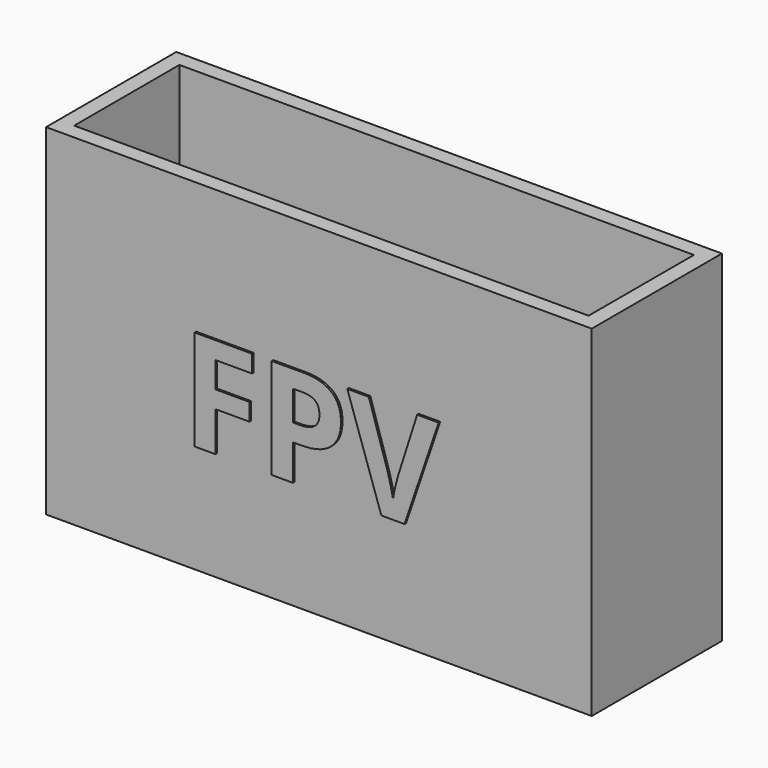
from build123d import *

# Parameters (mm, degrees)
F0_W         = 56
F0_H         = 16.7
F1_DEPTH     = 35
F2_T         = -1.6
F3_W         = 18.65
F3_H         = 13.5
F4_DEPTH     = 1.6
F5_TEXT_SIZE = 14.4269382064
F6_DEPTH     = 0.2


# Not quite as in the source:
# - Text() gives the source's letters only with a copy of the font that has no kerning and outlines rounded to 1/6400 em; it was checked with that copy


with BuildPart() as f1:
    # F0 (on Top) → F1 (new body)
    with BuildSketch(Plane.XY):
        Rectangle(F0_W, F0_H)
    extrude(amount=F1_DEPTH)

    # F2
    f2_openings = [f1.faces().sort_by_distance(p)[0] for p in [
        (0, 0, 35),
    ]]
    offset(amount=F2_T, openings=f2_openings)

    # F3 (on face) → F4 (cut, through all)
    with BuildSketch(Plane(origin=(0, 0, 0), x_dir=(1, 0, 0), z_dir=(0, 0, -1))):
        with Locations((16.825, 0)):
            Rectangle(F3_W, F3_H)
        with Locations((-16.825, 0)):
            Rectangle(F3_W, F3_H)
    extrude(amount=-F4_DEPTH, mode=Mode.SUBTRACT)

    # F5 (on face) → F6 (join)
    with BuildSketch(Plane.XZ.offset(8.35)):
        with Locations((-13.9068523422, 11.231337674)):
            Text('FPV', F5_TEXT_SIZE, font='Open Sans', font_style=FontStyle.BOLD, text_align=(TextAlign.LEFT, TextAlign.BOTTOM))
    extrude(amount=F6_DEPTH)


solid = f1.part
